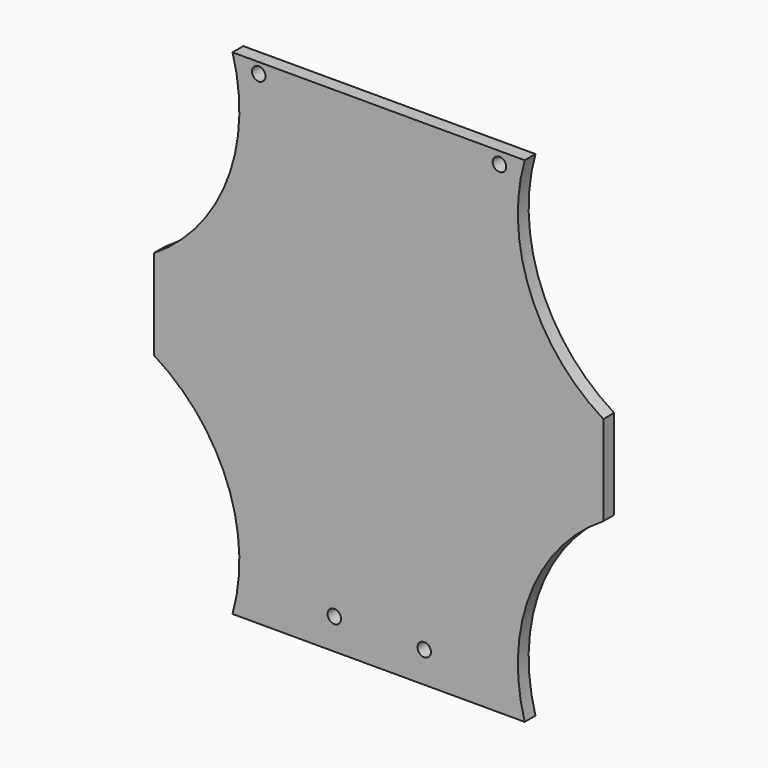
from build123d import *

# Parameters (mm, degrees)
F0_W      = 100
F0_H      = 110
F1_DEPTH  = 3
F3_DEPTH  = 25
F4_W      = 15
F4_H      = 6
F5_DEPTH  = 30
F6_R      = 3
F7_R      = 2.99999
F8_R      = 1.5
F9_DEPTH  = 25
F10_R     = 1.5
F11_DEPTH = 25


# Not quite as in the source:
# - a fillet or chamfer is up to 0.001 mm smaller than in the source, because OpenCascade refuses the exact size


with BuildPart() as f1:
    # F0 (on Front) → F1 (new body)
    with BuildSketch(Plane.XZ):
        with Locations((50, 55)):
            Rectangle(F0_W, F0_H)
    extrude(amount=F1_DEPTH)

    # F2 (on face) → F3 (cut)
    with BuildSketch(Plane.XZ.offset(3)):
        with BuildLine():
            Line((0, 110), (0, 65))
            ThreePointArc((0, 65), (16.3054104548, 84.5617848231), (17.5, 110))
            Line((17.5, 110), (0, 110))
        make_face()
        with BuildLine():
            Line((100, 110), (82.5, 110))
            ThreePointArc((82.5, 110), (83.6945895452, 84.5617848231), (100, 65))
            Line((100, 65), (100, 110))
        make_face()
        with BuildLine():
            ThreePointArc((100, 45), (83.6945895452, 25.4382151769), (82.5, 0))
            Line((82.5, 0), (100, 0))
            Line((100, 0), (100, 45))
        make_face()
        with BuildLine():
            Line((0, 45), (0, 0))
            Line((0, 0), (17.5, 0))
            ThreePointArc((17.5, 0), (16.3054104548, 25.4382151769), (0, 45))
        make_face()
    extrude(amount=-F3_DEPTH, mode=Mode.SUBTRACT)

    # F4 (on face) → F5 (join)
    with BuildSketch(Plane(origin=(0, 0, 0), x_dir=(-1, 0, 0), z_dir=(0, 1, 0))):
        with Locations((-50, 7)):
            Rectangle(F4_W, F4_H)
    extrude(amount=F5_DEPTH)

    # F6
    f6_edges = [f1.edges().sort_by_distance(p)[0] for p in [
        (50, 30, 4),
    ]]
    fillet(f6_edges, radius=F6_R)

    # F7 (radius 3 in the source; OpenCascade refuses exactly that, so slightly less here)
    f7_edges = [f1.edges().sort_by_distance(p)[0] for p in [
        (50, 30, 10),
    ]]
    fillet(f7_edges, radius=F7_R)

    # F8 (on face) → F9 (cut)
    with BuildSketch(Plane(origin=(0, 0, 0), x_dir=(-1, 0, 0), z_dir=(0, 1, 0))):
        with Locations((-40.1520836353, 6.8762069568)):
            Circle(F8_R)
        with Locations((-60.1520836353, 6.8762069568)):
            Circle(F8_R)
    extrude(amount=-F9_DEPTH, mode=Mode.SUBTRACT)

    # F10 (on face) → F11 (cut)
    with BuildSketch(Plane.XZ.offset(3)):
        with Locations((23.3403220773, 107.6833680272)):
            Circle(F10_R)
        with Locations((76.8845230341, 107.3717549443)):
            Circle(F10_R)
    extrude(amount=-F11_DEPTH, mode=Mode.SUBTRACT)


solid = f1.part
